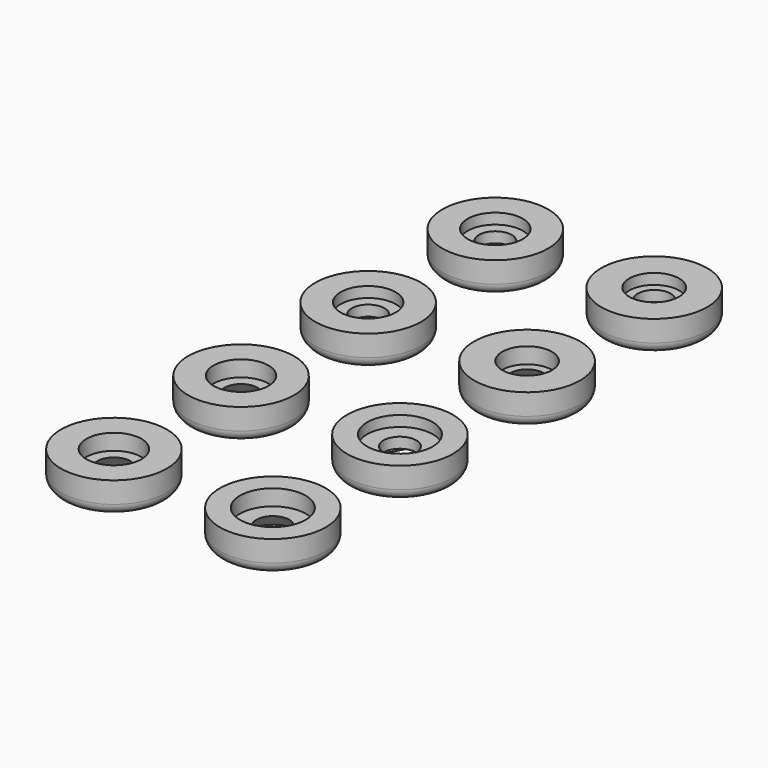
from build123d import *

# Parameters (mm, degrees)
F0_R       = 5
F0_R_2     = 1.55
F1_DEPTH   = 3
F2_R       = 2.6
F3_DEPTH   = 1.5
F4_R       = 2.6
F5_DEPTH   = 1.5
F6_R       = 2.6
F7_DEPTH   = 1
F8_R       = 2.6
F9_DEPTH   = 1
F10_R      = 3.1
F11_DEPTH  = 1.5
F12_R      = 3.1
F13_DEPTH  = 1
F14_R      = 2.35
F15_DEPTH  = 1.5
F16_R      = 2.35
F17_DEPTH  = 1
F19_DEPTH  = 1
F21_DEPTH  = 1
F23_DEPTH  = 1
F25_DEPTH  = 1
F26_SIZE   = 1.49999
F26_2_SIZE = 1.49999
F26_3_SIZE = 1.49999
F26_4_SIZE = 1.49999
F27_R      = 1
F27_2_R    = 1
F27_3_R    = 1
F27_4_R    = 1
F27_5_R    = 1
F27_6_R    = 1
F27_7_R    = 1
F27_8_R    = 1


# Not quite as in the source:
# - a fillet or chamfer is up to 0.001 mm smaller than in the source, because OpenCascade refuses the exact size


with BuildPart() as f1:
    # F0 (on Top) → F1 (new body)
    with BuildSketch(Plane.XY):
        with Locations((-31.0140149226, -17.6663821694)):
            Circle(F0_R)
        with Locations((-31.0140149226, -17.6663821694)):
            Circle(F0_R_2, mode=Mode.SUBTRACT)
    extrude(amount=F1_DEPTH)

    # F2 (on face) → F3 (cut)
    with BuildSketch(Plane.XY.offset(3)):
        with Locations((-31.0140149226, -17.6663821694)):
            Circle(F2_R)
    extrude(amount=-F3_DEPTH, mode=Mode.SUBTRACT)

    # F26#4 (size 1.5 in the source; OpenCascade refuses exactly that, so slightly less here)
    f26_4_edges = [f1.edges().sort_by_distance(p)[0] for p in [
        (-32.564015, -17.666382, 0),
    ]]
    chamfer(f26_4_edges, length=F26_4_SIZE)

    # F27
    f27_edges = [f1.edges().sort_by_distance(p)[0] for p in [
        (-36.014015, -17.666382, 0),
    ]]
    fillet(f27_edges, radius=F27_R)


with BuildPart() as f1b:
    # F0 (on Top) → F1, piece 2 (new body)
    with BuildSketch(Plane.XY):
        with Locations((-31.0140149226, -2.6663821694)):
            Circle(F0_R)
        with Locations((-31.0140149226, -2.6663821694)):
            Circle(F0_R_2, mode=Mode.SUBTRACT)
    extrude(amount=F1_DEPTH)

    # F4 (on face) → F5 (cut)
    with BuildSketch(Plane.XY.offset(3)):
        with Locations((-31.0140149226, -2.6663821694)):
            Circle(F4_R)
    extrude(amount=-F5_DEPTH, mode=Mode.SUBTRACT)

    # F26#3 (size 1.5 in the source; OpenCascade refuses exactly that, so slightly less here)
    f26_3_edges = [f1b.edges().sort_by_distance(p)[0] for p in [
        (-32.564015, -2.666382, 0),
    ]]
    chamfer(f26_3_edges, length=F26_3_SIZE)

    # F27#2
    f27_2_edges = [f1b.edges().sort_by_distance(p)[0] for p in [
        (-36.014015, -2.666382, 0),
    ]]
    fillet(f27_2_edges, radius=F27_2_R)


with BuildPart() as f1c:
    # F0 (on Top) → F1, piece 3 (new body)
    with BuildSketch(Plane.XY):
        with Locations((-31.0140149226, 12.3336178306)):
            Circle(F0_R)
        with Locations((-31.0140149226, 12.3336178306)):
            Circle(F0_R_2, mode=Mode.SUBTRACT)
    extrude(amount=F1_DEPTH)

    # F6 (on face) → F7 (cut)
    with BuildSketch(Plane.XY.offset(3)):
        with Locations((-31.0140149226, 12.3336178306)):
            Circle(F6_R)
    extrude(amount=-F7_DEPTH, mode=Mode.SUBTRACT)

    # F20 (on face) → F21 (cut)
    with BuildSketch(Plane(origin=(0, 0, 0), x_dir=(1, 0, 0), z_dir=(0, 0, -1))):
        Polygon((-31.0935447109, -15.7968063922), (-28.0545705444, -14.1340869284), (-27.9750407561, -10.6708983669), (-30.9344851344, -8.8704292691), (-33.9734593009, -10.5331487329), (-34.0529890891, -13.9963372944), align=None)
    extrude(amount=-F21_DEPTH, mode=Mode.SUBTRACT)

    # F27#6
    f27_6_edges = [f1c.edges().sort_by_distance(p)[0] for p in [
        (-36.014015, 12.333618, 0),
    ]]
    fillet(f27_6_edges, radius=F27_6_R)


with BuildPart() as f1d:
    # F0 (on Top) → F1, piece 4 (new body)
    with BuildSketch(Plane.XY):
        with Locations((-31.0140149226, 27.3336178306)):
            Circle(F0_R)
        with Locations((-31.0140149226, 27.3336178306)):
            Circle(F0_R_2, mode=Mode.SUBTRACT)
    extrude(amount=F1_DEPTH)

    # F8 (on face) → F9 (cut)
    with BuildSketch(Plane.XY.offset(3)):
        with Locations((-31.0140149226, 27.3336178306)):
            Circle(F8_R)
    extrude(amount=-F9_DEPTH, mode=Mode.SUBTRACT)

    # F18 (on face) → F19 (cut)
    with BuildSketch(Plane(origin=(0, 0, 0), x_dir=(1, 0, 0), z_dir=(0, 0, -1))):
        Polygon((-31.5034920511, -30.7629635613), (-28.2888529657, -29.4721903239), (-27.7993758372, -26.0428445932), (-30.5245377941, -23.9042720999), (-33.7391768795, -25.1950453374), (-34.228654008, -28.6243910681), align=None)
    extrude(amount=-F19_DEPTH, mode=Mode.SUBTRACT)

    # F27#7
    f27_7_edges = [f1d.edges().sort_by_distance(p)[0] for p in [
        (-36.014015, 27.333618, 0),
    ]]
    fillet(f27_7_edges, radius=F27_7_R)


with BuildPart() as f1e:
    # F0 (on Top) → F1, piece 5 (new body)
    with BuildSketch(Plane.XY):
        with Locations((-16.0140149226, -17.6663821694)):
            Circle(F0_R)
        with Locations((-16.0140149226, -17.6663821694)):
            Circle(F0_R_2, mode=Mode.SUBTRACT)
    extrude(amount=F1_DEPTH)

    # F10 (on face) → F11 (cut)
    with BuildSketch(Plane.XY.offset(3)):
        with Locations((-16.0140149226, -17.6663821694)):
            Circle(F10_R)
    extrude(amount=-F11_DEPTH, mode=Mode.SUBTRACT)

    # F26 (size 1.5 in the source; OpenCascade refuses exactly that, so slightly less here)
    f26_edges = [f1e.edges().sort_by_distance(p)[0] for p in [
        (-17.564015, -17.666382, 0),
    ]]
    chamfer(f26_edges, length=F26_SIZE)

    # F27#4
    f27_4_edges = [f1e.edges().sort_by_distance(p)[0] for p in [
        (-21.014015, -17.666382, 0),
    ]]
    fillet(f27_4_edges, radius=F27_4_R)


with BuildPart() as f1f:
    # F0 (on Top) → F1, piece 6 (new body)
    with BuildSketch(Plane.XY):
        with Locations((-16.0140149226, -2.6663821694)):
            Circle(F0_R)
        with Locations((-16.0140149226, -2.6663821694)):
            Circle(F0_R_2, mode=Mode.SUBTRACT)
    extrude(amount=F1_DEPTH)

    # F12 (on face) → F13 (cut)
    with BuildSketch(Plane.XY.offset(3)):
        with Locations((-16.0140149226, -2.6663821694)):
            Circle(F12_R)
    extrude(amount=-F13_DEPTH, mode=Mode.SUBTRACT)

    # F24 (on face) → F25 (cut)
    with BuildSketch(Plane(origin=(0, 0, 0), x_dir=(1, 0, 0), z_dir=(0, 0, -1))):
        Polygon((-17.7460657302, -0.3336178306), (-14.281964115, -0.3336178306), (-12.5499133075, 2.6663821694), (-14.281964115, 5.6663821694), (-17.7460657302, 5.6663821694), (-19.4781165378, 2.6663821694), align=None)
    extrude(amount=-F25_DEPTH, mode=Mode.SUBTRACT)

    # F27#3
    f27_3_edges = [f1f.edges().sort_by_distance(p)[0] for p in [
        (-21.014015, -2.666382, 0),
    ]]
    fillet(f27_3_edges, radius=F27_3_R)


with BuildPart() as f1g:
    # F0 (on Top) → F1, piece 7 (new body)
    with BuildSketch(Plane.XY):
        with Locations((-16.0140149226, 12.3336178306)):
            Circle(F0_R)
        with Locations((-16.0140149226, 12.3336178306)):
            Circle(F0_R_2, mode=Mode.SUBTRACT)
    extrude(amount=F1_DEPTH)

    # F14 (on face) → F15 (cut)
    with BuildSketch(Plane.XY.offset(3)):
        with Locations((-16.0140149226, 12.3336178306)):
            Circle(F14_R)
    extrude(amount=-F15_DEPTH, mode=Mode.SUBTRACT)

    # F26#2 (size 1.5 in the source; OpenCascade refuses exactly that, so slightly less here)
    f26_2_edges = [f1g.edges().sort_by_distance(p)[0] for p in [
        (-17.564015, 12.333618, 0),
    ]]
    chamfer(f26_2_edges, length=F26_2_SIZE)

    # F27#5
    f27_5_edges = [f1g.edges().sort_by_distance(p)[0] for p in [
        (-21.014015, 12.333618, 0),
    ]]
    fillet(f27_5_edges, radius=F27_5_R)


with BuildPart() as f1h:
    # F0 (on Top) → F1, piece 8 (new body)
    with BuildSketch(Plane.XY):
        with Locations((-16.0140149226, 27.3336178306)):
            Circle(F0_R)
        with Locations((-16.0140149226, 27.3336178306)):
            Circle(F0_R_2, mode=Mode.SUBTRACT)
    extrude(amount=F1_DEPTH)

    # F16 (on face) → F17 (cut)
    with BuildSketch(Plane.XY.offset(3)):
        with Locations((-16.0140149226, 27.3336178306)):
            Circle(F16_R)
    extrude(amount=-F17_DEPTH, mode=Mode.SUBTRACT)

    # F22 (on face) → F23 (cut)
    with BuildSketch(Plane(origin=(0, 0, 0), x_dir=(1, 0, 0), z_dir=(0, 0, -1))):
        Polygon((-17.0452971133, -30.6406492855), (-13.665682767, -29.8802501337), (-12.6344005763, -26.5732186789), (-14.9827327319, -24.0265863758), (-18.3623470782, -24.7869855276), (-19.393629269, -28.0940169824), align=None)
    extrude(amount=-F23_DEPTH, mode=Mode.SUBTRACT)

    # F27#8
    f27_8_edges = [f1h.edges().sort_by_distance(p)[0] for p in [
        (-21.014015, 27.333618, 0),
    ]]
    fillet(f27_8_edges, radius=F27_8_R)


solid = Compound([f1.part, f1b.part, f1c.part, f1d.part, f1e.part, f1f.part, f1g.part, f1h.part])
